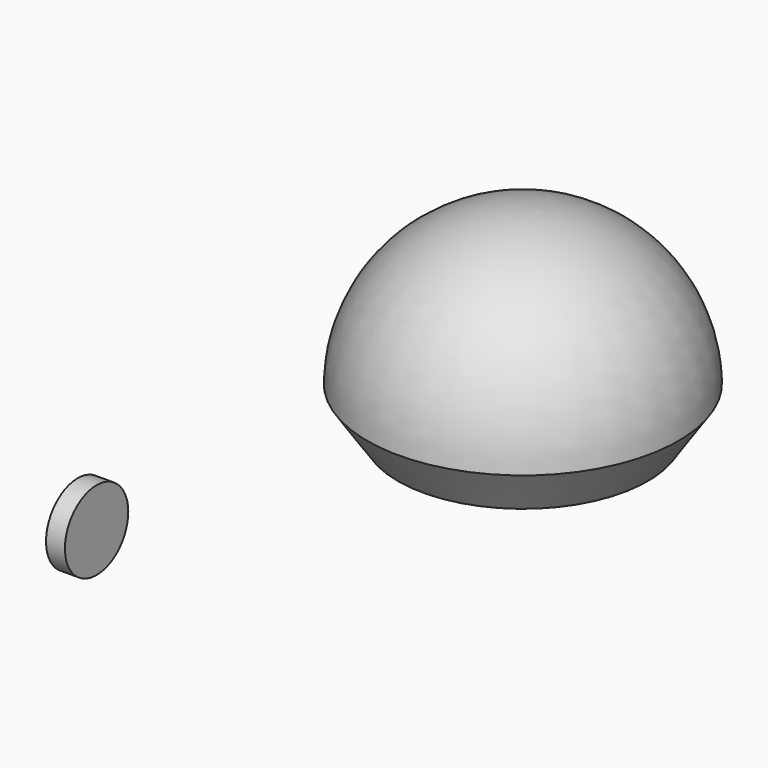
from build123d import *

# Parameters (mm, degrees)
F3_R     = 2.0966319248
F4_DEPTH = 1


# Not quite as in the source:
# - a fillet or chamfer that OpenCascade refuses, or shapes differently, is made with other operations: its cross-section is extruded or revolved along the edge and cut away or added


with BuildPart() as f1:
    # F0 (on Front) → F1 (revolve)
    with BuildSketch(Plane.XZ):
        with BuildLine():
            Line((-7.9164700583, 0), (0, 0))
            Line((0, 0), (0, 10.3605724871))
            ThreePointArc((0, 10.3605724871), (-6.5713696188, 7.1769714425), (-7.9164700583, 0))
        make_face()
    revolve(axis=Axis((0, 0, 5.1802862436), (0, 0, 1)))

    # F2: chamfer of 1 x 2 on 1 edges, made by hand

    # F2_s1 → F2_t2 (revolve, cut)
    with BuildSketch(Plane.XZ):
        with BuildLine():
            Line((-6.5703214108, -0.0663148568), (-8.2799279758, 2.467285589))
            Line((-8.2799279758, 2.467285589), (-8.3199215099, 2.4680047775))
            ThreePointArc((-8.3199215099, 2.4680047775), (-8.2103524238, 1.2192637953), (-7.9548909557, -0.0111281015))
            Line((-7.9548909557, -0.0111281015), (-7.9164700583, -0.04))
            ThreePointArc((-7.9164700583, -0.04), (-7.2433957345, -0.04), (-6.5703214108, -0.1063148568))
            Line((-6.5703214108, -0.1063148568), (-6.5703214108, -0.0663148568))
        make_face()
    revolve(axis=Axis((0, 0, 0), (0, 0, 1)), mode=Mode.SUBTRACT)


with BuildPart() as f4:
    # F3 (on Right) → F4 (new body)
    with BuildSketch(Plane.YZ):
        with Locations((-29.4634513557, 7.8704915941)):
            Circle(F3_R)
    extrude(amount=F4_DEPTH)


solid = Compound([f1.part, f4.part])
